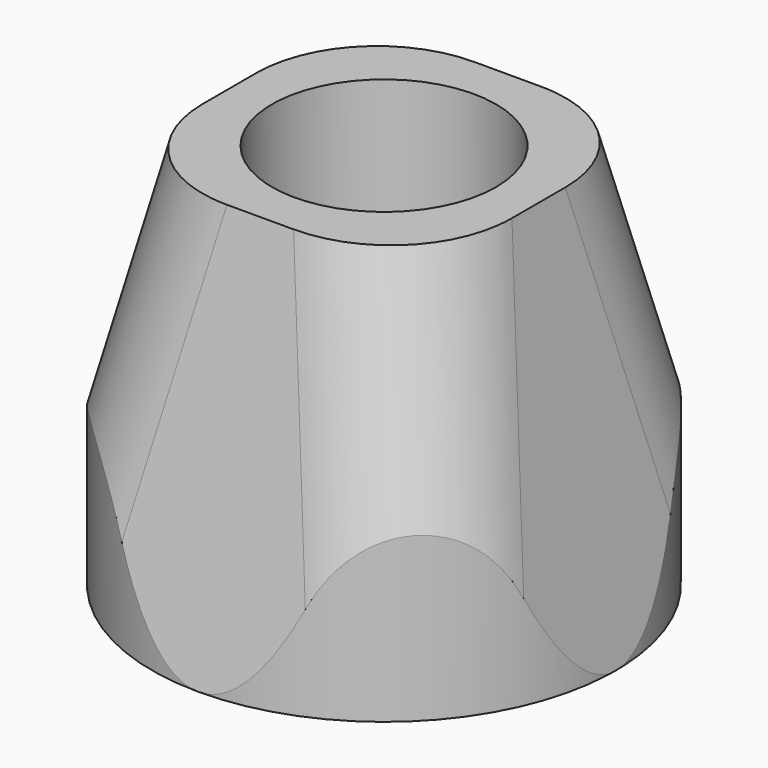
from build123d import *

# Parameters (mm, degrees)
F0_W        = 30
F0_H        = 30
F1_DEPTH    = 25
F2_R        = 7.25
F3_DEPTH    = 25
F4_SIZE2    = 24.99999
F4_SIZE     = 4.99999
F5_T1_DEPTH = 102.9607936575
F5_T3_DEPTH = 102.9607936575
F5_T5_DEPTH = 102.9607936575
F5_T7_DEPTH = 102.9607936575
F7_DEPTH    = 25
F8_R        = 11
F9_DEPTH    = 4


# Not quite as in the source:
# - a fillet or chamfer that OpenCascade refuses, or shapes differently, is made with other operations: its cross-section is extruded or revolved along the edge and cut away or added
# - a fillet or chamfer is up to 0.001 mm smaller than in the source, because OpenCascade refuses the exact size


with BuildPart() as f1:
    # F0 (on Top) → F1 (new body)
    with BuildSketch(Plane.XY):
        Rectangle(F0_W, F0_H)
    extrude(amount=F1_DEPTH)

    # F2 (on face) → F3 (cut)
    with BuildSketch(Plane.XY.offset(25)):
        Circle(F2_R)
    extrude(amount=-F3_DEPTH, mode=Mode.SUBTRACT)

    # F4 (size 5 and 25 in the source; OpenCascade refuses exactly that, so slightly less here)
    f4_edges = [f1.edges().sort_by_distance(p)[0] for p in [
        (15, 0, 25),
        (0, 15, 25),
        (-15, 0, 25),
        (0, -15, 25),
    ]]
    f4_side = f1.faces().sort_by_distance((14.575736, 0, 25))[0]
    chamfer(f4_edges, length=F4_SIZE, length2=F4_SIZE2, reference=f4_side)

    # F5: fillet of radius 8 on 4 edges, made by hand

    # F5_s2 → F5_t1 (cut)
    with BuildSketch(Plane(origin=(-7.5925826886, 7.5925826886, 37.9629741838), x_dir=(0.7071067812, 0.7071067812, 0), z_dir=(0.1924498046, -0.1924498046, -0.9622505627))):
        with BuildLine():
            ThreePointArc((5.5470023036, 15.0748135762), (0, 17.3102003677), (-5.5470023036, 15.0748135762))
            Line((-5.5470023036, 15.0748135762), (0, 20.4124196641))
            Line((0, 20.4124196641), (5.5470023036, 15.0748135762))
        make_face()
    extrude(amount=F5_T1_DEPTH, mode=Mode.SUBTRACT)

    # F5_s4 → F5_t3 (cut)
    with BuildSketch(Plane(origin=(-7.5925826886, -7.5925826886, 37.9629741838), x_dir=(-0.7071067812, 0.7071067812, 0), z_dir=(0.1924498046, 0.1924498046, -0.9622505627))):
        with BuildLine():
            ThreePointArc((-5.5470023036, 15.0748135762), (0, 17.3102003677), (5.5470023036, 15.0748135762))
            Line((5.5470023036, 15.0748135762), (0, 20.4124196641))
            Line((0, 20.4124196641), (-5.5470023036, 15.0748135762))
        make_face()
    extrude(amount=F5_T3_DEPTH, mode=Mode.SUBTRACT)

    # F5_s6 → F5_t5 (cut)
    with BuildSketch(Plane(origin=(7.5925826886, -7.5925826886, 37.9629741838), x_dir=(-0.7071067812, -0.7071067812, 0), z_dir=(-0.1924498046, 0.1924498046, -0.9622505627))):
        with BuildLine():
            ThreePointArc((-5.5470023036, 15.0748135762), (0, 17.3102003677), (5.5470023036, 15.0748135762))
            Line((5.5470023036, 15.0748135762), (0, 20.4124196641))
            Line((0, 20.4124196641), (-5.5470023036, 15.0748135762))
        make_face()
    extrude(amount=F5_T5_DEPTH, mode=Mode.SUBTRACT)

    # F5_s8 → F5_t7 (cut)
    with BuildSketch(Plane(origin=(7.5925826886, 7.5925826886, 37.9629741838), x_dir=(0.7071067812, -0.7071067812, 0), z_dir=(-0.1924498046, -0.1924498046, -0.9622505627))):
        with BuildLine():
            ThreePointArc((5.5470023036, 15.0748135762), (0, 17.3102003677), (-5.5470023036, 15.0748135762))
            Line((-5.5470023036, 15.0748135762), (0, 20.4124196641))
            Line((0, 20.4124196641), (5.5470023036, 15.0748135762))
        make_face()
    extrude(amount=F5_T7_DEPTH, mode=Mode.SUBTRACT)

    # F6 (on face) → F7 (cut)
    with BuildSketch(Plane(origin=(0, 0, 0), x_dir=(1, 0, 0), z_dir=(0, 0, -1))):
        with BuildLine():
            ThreePointArc((0, 15), (10.6066017178, 10.6066017178), (15, 0))
            Line((15, 0), (15, 7.1610644072))
            add(Edge.make_bspline(
                [(7.1610644072, 15), (14.9945107468, 14.9945107468), (15, 7.1610644072)],
                knots=[2.3761301528, 2.3761301528, 2.3761301528, 3.9070551544, 3.9070551544, 3.9070551544], degree=2, weights=[1, 0.7210619814, 1]))
            Line((7.1610644072, 15), (0, 15))
        make_face()
        with BuildLine():
            ThreePointArc((-15, 0), (-10.6066017178, 10.6066017178), (0, 15))
            Line((0, 15), (-7.1610644072, 15))
            add(Edge.make_bspline(
                [(-15, 7.1610644072), (-14.9945107468, 14.9945107468), (-7.1610644072, 15)],
                knots=[2.3761301528, 2.3761301528, 2.3761301528, 3.9070551544, 3.9070551544, 3.9070551544], degree=2, weights=[1, 0.7210619814, 1]))
            Line((-15, 7.1610644072), (-15, 0))
        make_face()
        with BuildLine():
            Line((-7.1610644072, -15), (0, -15))
            ThreePointArc((0, -15), (-10.6066017178, -10.6066017178), (-15, 0))
            Line((-15, 0), (-15, -7.1610644072))
            add(Edge.make_bspline(
                [(-7.1610644072, -15), (-14.9945107468, -14.9945107468), (-15, -7.1610644072)],
                knots=[2.3761301528, 2.3761301528, 2.3761301528, 3.9070551544, 3.9070551544, 3.9070551544], degree=2, weights=[1, 0.7210619814, 1]))
        make_face()
        with BuildLine():
            Line((15, -7.1610644072), (15, 0))
            ThreePointArc((15, 0), (10.6066017178, -10.6066017178), (0, -15))
            Line((0, -15), (7.1610644072, -15))
            add(Edge.make_bspline(
                [(15, -7.1610644072), (14.9945107468, -14.9945107468), (7.1610644072, -15)],
                knots=[2.3761301528, 2.3761301528, 2.3761301528, 3.9070551544, 3.9070551544, 3.9070551544], degree=2, weights=[1, 0.7210619814, 1]))
        make_face()
    extrude(amount=-F7_DEPTH, mode=Mode.SUBTRACT)

    # F8 (on face) → F9 (cut)
    with BuildSketch(Plane(origin=(0, 0, 0), x_dir=(1, 0, 0), z_dir=(0, 0, -1))):
        Circle(F8_R)
    extrude(amount=-F9_DEPTH, mode=Mode.SUBTRACT)


solid = f1.part
